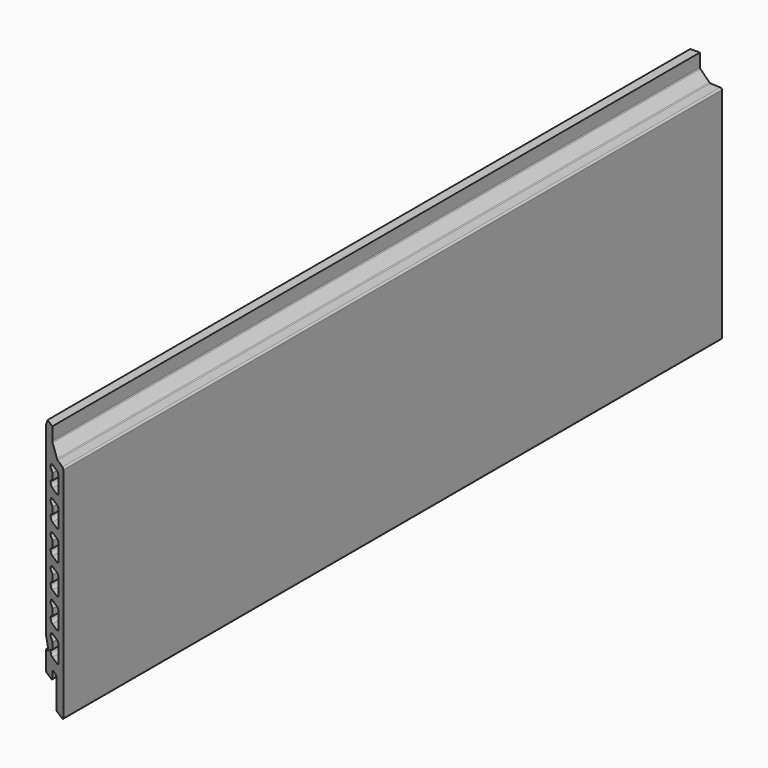
from build123d import *

# Parameters (mm, degrees)
F1_DEPTH      = 711.2
F3_DEPTH      = 711.2
F5_DEPTH      = 106.0997464
F5_DEPTH_BACK = 106.0997464


# Not quite as in the source:
# - ends of sketch curves that miss each other by under 0.0002 mm in the source are joined


with BuildPart() as f1:
    # F0 (on Front) → F1 (new body)
    with BuildSketch(Plane.XZ):
        with BuildLine():
            ThreePointArc((-14.9999680608, -58.9985104), (-14.96444377, -59.322873513), (-14.8595551032, -59.6318585804))
            Line((-14.8595551032, -59.6318585804), (-11.0988328608, -67.6967912))
            ThreePointArc((-11.0988328608, -67.6967912), (-11.1617050028, -68.655791158), (-12.004294, -69.1180454046))
            Line((-12.004294, -69.1180454046), (-14.0009118, -69.1180736))
            ThreePointArc((-14.0009118, -69.1180736), (-14.707352628, -69.410690972), (-14.99997, -70.1171318))
            Line((-14.99997, -70.1171318), (-14.99997, -85.599397))
            ThreePointArc((-14.99997, -85.599397), (-14.5606310505, -86.6600550505), (-13.499973, -87.099394))
            Line((-13.499973, -87.099394), (-5.5003446, -87.099394))
            ThreePointArc((-5.5003446, -87.099394), (-4.4396865495, -86.6600550505), (-4.0003476, -85.599397))
            Line((-4.0003476, -85.599397), (-4.0003476, -80.5996356))
            ThreePointArc((-4.0003476, -80.5996356), (-3.5610086505, -79.5389775495), (-2.5003506, -79.0996386))
            Line((-2.5003506, -79.0996386), (1.4838426, -79.0996386))
            ThreePointArc((1.4838426, -79.0996386), (2.5445365709, -79.5390134712), (2.9838395966, -80.5997372))
            Line((2.9838395966, -80.5997372), (2.98196, -104.5986224))
            ThreePointArc((2.98196, -104.5986224), (3.4212540492, -105.6593625482), (4.481957, -106.0987464))
            Line((4.481957, -106.0987464), (13.499973, -106.0987464))
            ThreePointArc((13.499973, -106.0987464), (14.5606310505, -105.6594074505), (14.99997, -104.5987494))
            Line((14.99997, -104.5987494), (14.99997, 83.7761342))
            ThreePointArc((14.99997, 83.7761342), (14.5844487053, 84.8124273268), (13.5680958768, 85.2745834897))
            Line((13.5680958768, 85.2745834897), (5.104384, 85.6592902))
            ThreePointArc((5.104384, 85.6592902), (4.5671403109, 85.7853117853), (4.1118233495, 86.0970797495))
            Line((4.1118233495, 86.0970797495), (-3.5610038, 93.7699166))
            ThreePointArc((-3.5610038, 93.7699166), (-3.8861671271, 94.2565457995), (-4.0003476, 94.8305698))
            Line((-4.0003476, 94.8305698), (-4.0003476, 106.0987464))
            Line((-4.0003476, 106.0987464), (-12.3105164, 106.0987464))
            Line((-12.3105164, 106.0987464), (-14.99997, 101.2086876))
            Line((-14.99997, 101.2086876), (-14.9999680608, -58.9985104))
        make_face()
    extrude(amount=F1_DEPTH)

    # F2 (on Front) → F3 (cut)
    with BuildSketch(Plane.XZ):
        with BuildLine():
            ThreePointArc((-5.49529, -31.195264), (-4.4346319495, -31.6346029495), (-3.995293, -32.695261))
            Line((-3.995293, -32.695261), (-3.995293, -37.695251))
            ThreePointArc((-3.995293, -37.695251), (-4.4346319495, -38.7559090505), (-5.49529, -39.195248))
            Line((-5.49529, -39.195248), (-5.499989, -39.195248))
            ThreePointArc((-5.499989, -39.195248), (-6.5606470505, -39.6345869495), (-6.999986, -40.695245))
            Line((-6.999986, -40.695245), (-6.999986, -41.195244))
            ThreePointArc((-6.999986, -41.195244), (-6.1213081009, -43.3165601009), (-3.999992, -44.195238))
            Line((-3.999992, -44.195238), (3.999992, -44.195238))
            ThreePointArc((3.999992, -44.195238), (6.1213081009, -43.3165601009), (6.999986, -41.195244))
            Line((6.999986, -41.195244), (6.999986, -29.195268))
            ThreePointArc((6.999986, -29.195268), (6.1213081009, -27.0739518991), (3.999992, -26.195274))
            Line((3.999992, -26.195274), (-3.999992, -26.195274))
            ThreePointArc((-3.999992, -26.195274), (-6.1213081009, -27.0739518991), (-6.999986, -29.195268))
            Line((-6.999986, -29.195268), (-6.999986, -29.695267))
            ThreePointArc((-6.999986, -29.695267), (-6.5606470505, -30.7559250505), (-5.499989, -31.195264))
            Line((-5.499989, -31.195264), (-5.49529, -31.195264))
        make_face()
        with BuildLine():
            ThreePointArc((-5.49529, -56.595264), (-4.4346319495, -57.0346029495), (-3.995293, -58.095261))
            Line((-3.995293, -58.095261), (-3.995293, -63.095251))
            ThreePointArc((-3.995293, -63.095251), (-4.4346319495, -64.1559090505), (-5.49529, -64.595248))
            Line((-5.49529, -64.595248), (-5.499989, -64.595248))
            ThreePointArc((-5.499989, -64.595248), (-6.5606470505, -65.0345869495), (-6.999986, -66.095245))
            Line((-6.999986, -66.095245), (-6.999986, -66.595244))
            ThreePointArc((-6.999986, -66.595244), (-6.1213081009, -68.7165601009), (-3.999992, -69.595238))
            Line((-3.999992, -69.595238), (0, -69.595238))
            Line((0, -69.595238), (3.999992, -69.595238))
            ThreePointArc((3.999992, -69.595238), (6.1213081009, -68.7165601009), (6.999986, -66.595244))
            Line((6.999986, -66.595244), (6.999986, -54.595268))
            ThreePointArc((6.999986, -54.595268), (6.1213081009, -52.4739518991), (3.999992, -51.595274))
            Line((3.999992, -51.595274), (-3.999992, -51.595274))
            ThreePointArc((-3.999992, -51.595274), (-6.1213081009, -52.4739518991), (-6.999986, -54.595268))
            Line((-6.999986, -54.595268), (-6.999986, -55.095267))
            ThreePointArc((-6.999986, -55.095267), (-6.5606470505, -56.1559250505), (-5.499989, -56.595264))
            Line((-5.499989, -56.595264), (-5.49529, -56.595264))
        make_face()
        with BuildLine():
            ThreePointArc((-5.49529, -5.3953664), (-4.4346319495, -5.8347053495), (-3.995293, -6.8953634))
            Line((-3.995293, -6.8953634), (-3.995293, -11.8953534))
            ThreePointArc((-3.995293, -11.8953534), (-4.4346319495, -12.9560114505), (-5.49529, -13.3953504))
            Line((-5.49529, -13.3953504), (-5.499989, -13.3953504))
            ThreePointArc((-5.499989, -13.3953504), (-6.5606470505, -13.8346893495), (-6.999986, -14.8953474))
            Line((-6.999986, -14.8953474), (-6.999986, -15.3953464))
            ThreePointArc((-6.999986, -15.3953464), (-6.1213081009, -17.5166625009), (-3.999992, -18.3953404))
            Line((-3.999992, -18.3953404), (3.999992, -18.3953404))
            ThreePointArc((3.999992, -18.3953404), (6.1213081009, -17.5166625009), (6.999986, -15.3953464))
            Line((6.999986, -15.3953464), (6.999986, -3.3953704))
            ThreePointArc((6.999986, -3.3953704), (6.1213081009, -1.2740542991), (3.999992, -0.3953764))
            Line((3.999992, -0.3953764), (-3.999992, -0.3953764))
            ThreePointArc((-3.999992, -0.3953764), (-6.1213081009, -1.2740542991), (-6.999986, -3.3953704))
            Line((-6.999986, -3.3953704), (-6.999986, -3.8953694))
            ThreePointArc((-6.999986, -3.8953694), (-6.5606470505, -4.9560274505), (-5.499989, -5.3953664))
            Line((-5.499989, -5.3953664), (-5.49529, -5.3953664))
        make_face()
        with BuildLine():
            Line((-5.499989, 20.4015086), (-5.49529, 20.4015086))
            ThreePointArc((-5.49529, 20.4015086), (-4.4346319495, 19.9621696505), (-3.995293, 18.9015116))
            Line((-3.995293, 18.9015116), (-3.995293, 13.9015216))
            ThreePointArc((-3.995293, 13.9015216), (-4.4346319495, 12.8408635495), (-5.49529, 12.4015246))
            Line((-5.49529, 12.4015246), (-5.499989, 12.4015246))
            ThreePointArc((-5.499989, 12.4015246), (-6.5606470505, 11.9621856505), (-6.999986, 10.9015276))
            Line((-6.999986, 10.9015276), (-6.999986, 10.4015286))
            ThreePointArc((-6.999986, 10.4015286), (-6.1213081009, 8.2802124991), (-3.999992, 7.4015346))
            Line((-3.999992, 7.4015346), (3.999992, 7.4015346))
            ThreePointArc((3.999992, 7.4015346), (6.1213081009, 8.2802124991), (6.999986, 10.4015286))
            Line((6.999986, 10.4015286), (6.999986, 22.4015046))
            ThreePointArc((6.999986, 22.4015046), (6.1213081009, 24.5228207009), (3.999992, 25.4014986))
            Line((3.999992, 25.4014986), (-3.999992, 25.4014986))
            ThreePointArc((-3.999992, 25.4014986), (-6.1213081009, 24.5228207009), (-6.999986, 22.4015046))
            Line((-6.999986, 22.4015046), (-6.999986, 21.9015056))
            ThreePointArc((-6.999986, 21.9015056), (-6.5606470505, 20.8408475495), (-5.499989, 20.4015086))
        make_face()
        with BuildLine():
            Line((-5.499989, 46.1983836), (-5.49529, 46.1983836))
            ThreePointArc((-5.49529, 46.1983836), (-4.4346319495, 45.7590446505), (-3.995293, 44.6983866))
            Line((-3.995293, 44.6983866), (-3.995293, 39.6983966))
            ThreePointArc((-3.995293, 39.6983966), (-4.4346319495, 38.6377385495), (-5.49529, 38.1983996))
            Line((-5.49529, 38.1983996), (-5.499989, 38.1983996))
            ThreePointArc((-5.499989, 38.1983996), (-6.5606470505, 37.7590606505), (-6.999986, 36.6984026))
            Line((-6.999986, 36.6984026), (-6.999986, 36.1984036))
            ThreePointArc((-6.999986, 36.1984036), (-6.1213081009, 34.0770874991), (-3.999992, 33.1984096))
            Line((-3.999992, 33.1984096), (3.999992, 33.1984096))
            ThreePointArc((3.999992, 33.1984096), (6.1213081009, 34.0770874991), (6.999986, 36.1984036))
            Line((6.999986, 36.1984036), (6.999986, 48.1983796))
            ThreePointArc((6.999986, 48.1983796), (6.1213081009, 50.3196957009), (3.999992, 51.1983736))
            Line((3.999992, 51.1983736), (-3.999992, 51.1983736))
            ThreePointArc((-3.999992, 51.1983736), (-6.1213081009, 50.3196957009), (-6.999986, 48.1983796))
            Line((-6.999986, 48.1983796), (-6.999986, 47.6983806))
            ThreePointArc((-6.999986, 47.6983806), (-6.5606470505, 46.6377225495), (-5.499989, 46.1983836))
        make_face()
        with BuildLine():
            Line((-5.499989, 71.9952586), (-5.49529, 71.9952586))
            ThreePointArc((-5.49529, 71.9952586), (-4.4346319495, 71.5559196505), (-3.995293, 70.4952616))
            Line((-3.995293, 70.4952616), (-3.995293, 65.4952716))
            ThreePointArc((-3.995293, 65.4952716), (-4.4346319495, 64.4346135495), (-5.49529, 63.9952746))
            Line((-5.49529, 63.9952746), (-5.499989, 63.9952746))
            ThreePointArc((-5.499989, 63.9952746), (-6.5606470505, 63.5559356505), (-6.999986, 62.4952776))
            Line((-6.999986, 62.4952776), (-6.999986, 61.9952786))
            ThreePointArc((-6.999986, 61.9952786), (-6.1213081009, 59.8739624991), (-3.999992, 58.9952846))
            Line((-3.999992, 58.9952846), (3.999992, 58.9952846))
            ThreePointArc((3.999992, 58.9952846), (6.1213081009, 59.8739624991), (6.999986, 61.9952786))
            Line((6.999986, 61.9952786), (6.999986, 73.9952546))
            ThreePointArc((6.999986, 73.9952546), (6.1213081009, 76.1165707009), (3.999992, 76.9952486))
            Line((3.999992, 76.9952486), (-3.999992, 76.9952486))
            ThreePointArc((-3.999992, 76.9952486), (-6.1213081009, 76.1165707009), (-6.999986, 73.9952546))
            Line((-6.999986, 73.9952546), (-6.999986, 73.4952556))
            ThreePointArc((-6.999986, 73.4952556), (-6.5606470505, 72.4345975495), (-5.499989, 71.9952586))
        make_face()
    extrude(amount=F3_DEPTH, mode=Mode.SUBTRACT)

    # F4 (on Top) → F5 (cut, two sides)
    with BuildSketch(Plane.XY) as f5_sk:
        Polygon((-15.0409955531, -711.2733125687), (15.1156112552, -711.2733125687), (-15.0409955531, -692.2233125687), align=None)
    extrude(amount=F5_DEPTH, mode=Mode.SUBTRACT)
    extrude(f5_sk.sketch, amount=-F5_DEPTH_BACK, mode=Mode.SUBTRACT)


solid = f1.part
